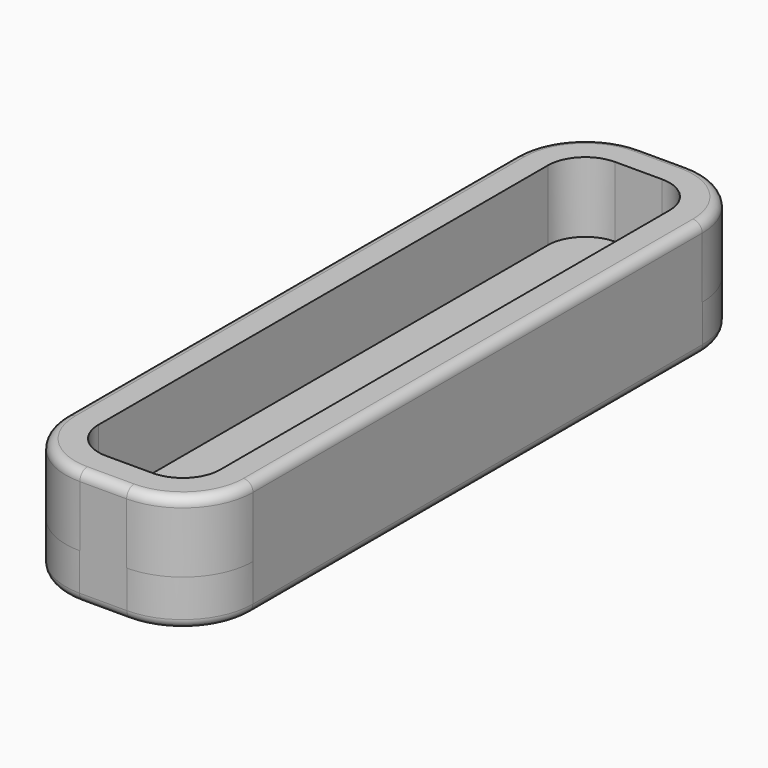
from build123d import *

# Parameters (mm, degrees)
F0_W         = 40
F0_H         = 150
F11_DEPTH    = 25
F1_R         = 15
F2_R         = 15
F3_R         = 15
F5_T         = -7
F6_DEPTH     = 10
F12_T1_DEPTH = 84.9995000017
F7_R         = 2


# Not quite as in the source:
# - a fillet or chamfer that OpenCascade refuses, or shapes differently, is made with other operations: its cross-section is extruded or revolved along the edge and cut away or added
# - a feature of the source that left no trace in its solid (it failed there, or was rolled back) is left out


with BuildPart() as f11:
    # F0 (on Top) → F11 (new body)
    with BuildSketch(Plane.XY):
        Rectangle(F0_W, F0_H)
    extrude(amount=F11_DEPTH)

    # F1
    f1_edges = [f11.edges().sort_by_distance(p)[0] for p in [
        (20, -75, 12.5),
    ]]
    fillet(f1_edges, radius=F1_R)

    # F2
    f2_edges = [f11.edges().sort_by_distance(p)[0] for p in [
        (-20, -75, 12.5),
    ]]
    fillet(f2_edges, radius=F2_R)

    # F3
    f3_edges = [f11.edges().sort_by_distance(p)[0] for p in [
        (-20, 75, 12.5),
        (20, 75, 12.5),
    ]]
    fillet(f3_edges, radius=F3_R)

    # F5
    f5_openings = [f11.faces().sort_by_distance(p)[0] for p in [
        (0, 0, 25),
    ]]
    offset(amount=F5_T, openings=f5_openings)

    # F0 (on Top) → F6 (join)
    with BuildSketch(Plane.XY):
        Rectangle(F0_W, F0_H)
    extrude(amount=F6_DEPTH)

    # F12: fillet of radius 15 on 4 edges, made by hand

    # F12_s2 → F12_t1 (cut)
    with BuildSketch(Plane.XY.offset(-37.4997500008)):
        with BuildLine():
            ThreePointArc((20.0001, -60.0001), (15.6067017178, -70.6067017178), (5.0001, -75.0001))
            Line((5.0001, -75.0001), (5.0001, -75.3001))
            ThreePointArc((5.0001, -75.3001), (12.50005, -75.3), (20, -75.3))
            Line((20, -75.3), (20.3, -75))
            ThreePointArc((20.3, -75), (20.3, -67.50005), (20.3001, -60.0001))
            Line((20.3001, -60.0001), (20.0001, -60.0001))
        make_face()
        with BuildLine():
            ThreePointArc((-5.0001, -75.0001), (-15.6067017178, -70.6067017178), (-20.0001, -60.0001))
            Line((-20.0001, -60.0001), (-20.3001, -60.0001))
            ThreePointArc((-20.3001, -60.0001), (-20.3, -67.50005), (-20.3, -75))
            Line((-20.3, -75), (-20, -75.3))
            ThreePointArc((-20, -75.3), (-12.50005, -75.3), (-5.0001, -75.3001))
            Line((-5.0001, -75.3001), (-5.0001, -75.0001))
        make_face()
        with BuildLine():
            ThreePointArc((5.0001, 75.0001), (15.6067017178, 70.6067017178), (20.0001, 60.0001))
            Line((20.0001, 60.0001), (20.3001, 60.0001))
            ThreePointArc((20.3001, 60.0001), (20.3, 67.50005), (20.3, 75))
            Line((20.3, 75), (20, 75.3))
            ThreePointArc((20, 75.3), (12.50005, 75.3), (5.0001, 75.3001))
            Line((5.0001, 75.3001), (5.0001, 75.0001))
        make_face()
        with BuildLine():
            ThreePointArc((-5.0001, 75.0001), (-15.6067017178, 70.6067017178), (-20.0001, 60.0001))
            Line((-20.0001, 60.0001), (-20.3001, 60.0001))
            ThreePointArc((-20.3001, 60.0001), (-20.3, 67.50005), (-20.3, 75))
            Line((-20.3, 75), (-20, 75.3))
            ThreePointArc((-20, 75.3), (-12.50005, 75.3), (-5.0001, 75.3001))
            Line((-5.0001, 75.3001), (-5.0001, 75.0001))
        make_face()
    extrude(amount=F12_T1_DEPTH, mode=Mode.SUBTRACT)

    # F7
    f7_edges = [f11.edges().sort_by_distance(p)[0] for p in [
        (20, 0, 0),
        (-20, 0, 0),
        (-15.606702, 70.606702, 0),
        (0, 75, 0),
        (15.606702, 70.606702, 0),
        (15.606702, -70.606702, 0),
        (0, -75, 0),
        (-15.606702, -70.606702, 0),
        (-20, 0, 25),
        (0, 75, 25),
        (20, 0, 25),
        (0, -75, 25),
        (-15.606602, -70.606602, 25),
        (15.606602, -70.606602, 25),
        (15.606602, 70.606602, 25),
        (-15.606602, 70.606602, 25),
    ]]
    fillet(f7_edges, radius=F7_R)


solid = f11.part
